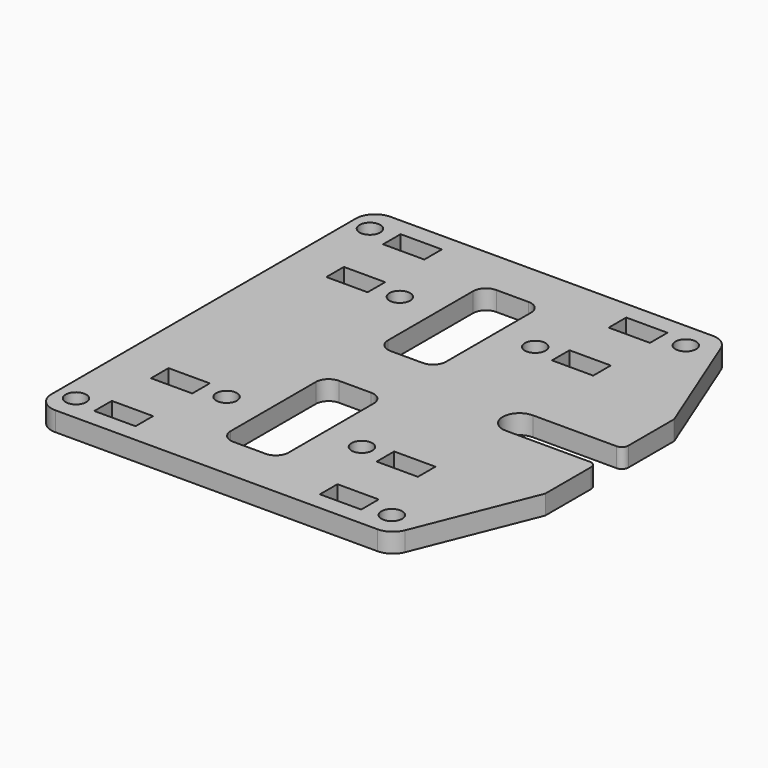
from build123d import *

# Parameters (mm, degrees)
F0_R     = 1.60312
F0_W     = 6.4
F0_H     = 3.4
F1_DEPTH = 3


# Not quite as in the source:
# - ends of sketch curves that miss each other by under 0.0002 mm in the source are joined


with BuildPart() as f1:
    # F0 (on Top) → F1 (new body)
    with BuildSketch(Plane.XY):
        with BuildLine():
            ThreePointArc((17.5, -2.6), (14.9, 0), (17.5, 2.6))
            Line((17.5, 2.6), (30.5, 2.6))
            ThreePointArc((30.5, 2.6), (31.2071067812, 2.8928932188), (31.5, 3.6))
            Line((31.5, 3.6), (31.5, 12.5))
            Line((31.5, 12.5), (24.2543, 30.6142))
            ThreePointArc((24.2543, 30.6142), (23.1507874279, 31.9842016914), (21.468901, 32.5))
            Line((21.468901, 32.5), (-28.5, 32.5))
            ThreePointArc((-28.5, 32.5), (-30.6213203436, 31.6213203436), (-31.5, 29.5))
            Line((-31.5, 29.5), (-31.5, -29.5))
            ThreePointArc((-31.5, -29.5), (-30.6213203436, -31.6213203436), (-28.5, -32.5))
            Line((-28.5, -32.5), (21.468901, -32.5))
            ThreePointArc((21.468901, -32.5), (23.1507874279, -31.9842016914), (24.2543310727, -30.6141720291))
            Line((24.2543310727, -30.6141720291), (31.5, -12.5))
            Line((31.5, -12.5), (31.5, -3.6))
            ThreePointArc((31.5, -3.6), (31.2071067812, -2.8928932188), (30.5, -2.6))
            Line((30.5, -2.6), (17.5, -2.6))
        make_face()
        with Locations((-28.5, -28.5)):
            Circle(F0_R, mode=Mode.SUBTRACT)
        with Locations((-21.5, -28)):
            Rectangle(F0_W, F0_H, mode=Mode.SUBTRACT)
        with Locations((-21.5, -17)):
            Rectangle(F0_W, F0_H, mode=Mode.SUBTRACT)
        with Locations((-14.5, -16.8)):
            Circle(F0_R, mode=Mode.SUBTRACT)
        with BuildLine():
            ThreePointArc((0.5, -23.5), (-0.0857864376, -24.9142135624), (-1.5, -25.5))
            Line((-1.5, -25.5), (-6.5, -25.5))
            ThreePointArc((-6.5, -25.5), (-7.9142135624, -24.9142135624), (-8.5, -23.5))
            Line((-8.5, -23.5), (-8.5, -7))
            ThreePointArc((-8.5, -7), (-7.9142135624, -5.5857864376), (-6.5, -5))
            Line((-6.5, -5), (-1.5, -5))
            ThreePointArc((-1.5, -5), (-0.0857864376, -5.5857864376), (0.5, -7))
            Line((0.5, -7), (0.5, -23.5))
        make_face(mode=Mode.SUBTRACT)
        with Locations((13.5, -28)):
            Rectangle(F0_W, F0_H, mode=Mode.SUBTRACT)
        with Locations((6.5, -16.8)):
            Circle(F0_R, mode=Mode.SUBTRACT)
        with Locations((13.5, -17)):
            Rectangle(F0_W, F0_H, mode=Mode.SUBTRACT)
        with Locations((20.5, -28.5)):
            Circle(F0_R, mode=Mode.SUBTRACT)
        with BuildLine():
            ThreePointArc((-1.5, 25.5), (-0.0857864376, 24.9142135624), (0.5, 23.5))
            Line((0.5, 23.5), (0.5, 7))
            ThreePointArc((0.5, 7), (-0.0857864376, 5.5857864376), (-1.5, 5))
            Line((-1.5, 5), (-6.5, 5))
            ThreePointArc((-6.5, 5), (-7.9142135624, 5.5857864376), (-8.5, 7))
            Line((-8.5, 7), (-8.5, 23.5))
            ThreePointArc((-8.5, 23.5), (-7.9142135624, 24.9142135624), (-6.5, 25.5))
            Line((-6.5, 25.5), (-1.5, 25.5))
        make_face(mode=Mode.SUBTRACT)
        with Locations((-21.5, 17)):
            Rectangle(F0_W, F0_H, mode=Mode.SUBTRACT)
        with Locations((-28.5, 28.5)):
            Circle(F0_R, mode=Mode.SUBTRACT)
        with Locations((-21.5, 28)):
            Rectangle(F0_W, F0_H, mode=Mode.SUBTRACT)
        with Locations((-14.5, 16.8)):
            Circle(F0_R, mode=Mode.SUBTRACT)
        with Locations((6.5, 16.8)):
            Circle(F0_R, mode=Mode.SUBTRACT)
        with Locations((13.5, 17)):
            Rectangle(F0_W, F0_H, mode=Mode.SUBTRACT)
        with Locations((13.5, 28)):
            Rectangle(F0_W, F0_H, mode=Mode.SUBTRACT)
        with Locations((20.5, 28.5)):
            Circle(F0_R, mode=Mode.SUBTRACT)
    extrude(amount=F1_DEPTH)


solid = f1.part
